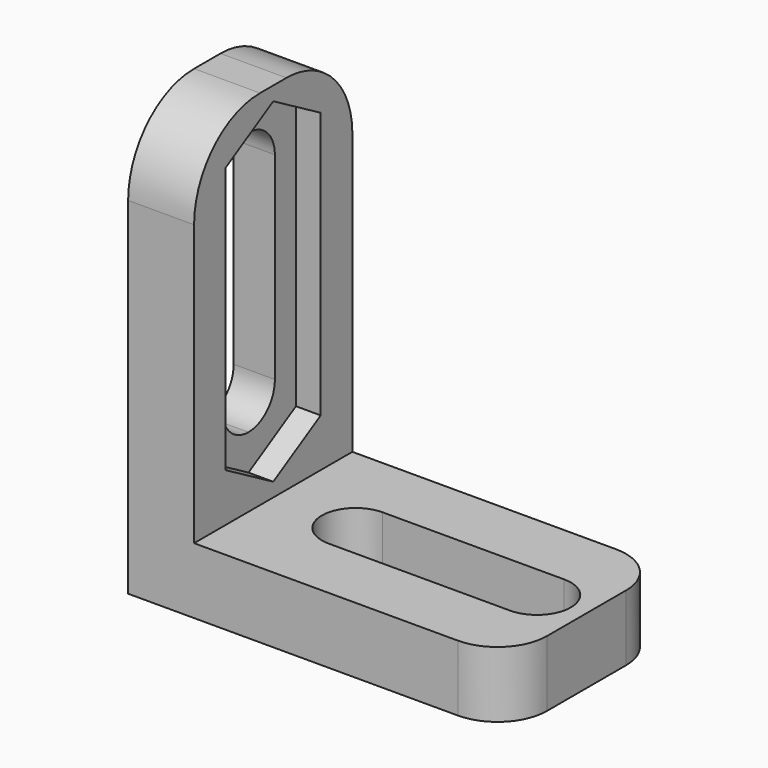
from build123d import *

# Parameters (mm, degrees)
F1_DEPTH = 4
F2_W     = 4
F2_H     = 12
F3_DEPTH = 22
F5_DEPTH = 25
F7_DEPTH = 1.5
F8_R     = 5


# Not quite as in the source:
# - a feature names something its author has since deleted; it is built from what else it names


with BuildPart() as f1:
    # F0 (on Top) → F1 (new body)
    with BuildSketch(Plane.XY):
        with BuildLine():
            ThreePointArc((0, -3), (-0.8786796564, -0.8786796564), (-3, 0))
            Line((-3, 0), (-23, 0))
            Line((-23, 0), (-23, -12))
            Line((-23, -12), (-3, -12))
            ThreePointArc((-3, -12), (-0.8786796564, -11.1213203436), (0, -9))
            Line((0, -9), (0, -3))
        make_face()
        with BuildLine():
            ThreePointArc((-3, -3.95), (-0.95, -6), (-3, -8.05))
            Line((-3, -8.05), (-14, -8.05))
            ThreePointArc((-14, -8.05), (-16.05, -6), (-14, -3.95))
            Line((-14, -3.95), (-3, -3.95))
        make_face(mode=Mode.SUBTRACT)
    extrude(amount=F1_DEPTH)

    # F2 (on face) → F3 (join)
    with BuildSketch(Plane.XY.offset(4)):
        with Locations((-21, -6)):
            Rectangle(F2_W, F2_H)
    extrude(amount=F3_DEPTH)

    # F4 (on face) → F5 (cut)
    with BuildSketch(Plane(origin=(-23, 0, 0), x_dir=(0, -1, 0), z_dir=(-1, 0, 0))):
        with BuildLine():
            Line((4, 21), (4, 9))
            ThreePointArc((4, 9), (4.5857864376, 7.5857864376), (6, 7))
            ThreePointArc((6, 7), (7.4142135624, 7.5857864376), (8, 9))
            Line((8, 9), (8, 21))
            ThreePointArc((8, 21), (7.4142135624, 22.4142135624), (6, 23))
            ThreePointArc((6, 23), (4.5857864376, 22.4142135624), (4, 21))
        make_face()
    extrude(amount=-F5_DEPTH, mode=Mode.SUBTRACT)

    # F6 (on face) → F7 (cut)
    with BuildSketch(Plane.YZ.offset(-19)):
        Polygon((-6, 4.8430780618), (-2.4, 6.9215390309), (-2.4, 23.0784609691), (-6, 25.1569219382), (-9.6, 23.0784609691), (-9.6, 6.9215390309), align=None)
        with BuildLine():
            ThreePointArc((-8, 21), (-6, 23), (-4, 21))
            Line((-4, 21), (-4, 9))
            ThreePointArc((-4, 9), (-6, 7), (-8, 9))
            Line((-8, 9), (-8, 21))
        make_face(mode=Mode.SUBTRACT)
    extrude(amount=-F7_DEPTH, mode=Mode.SUBTRACT)

    # F8
    f8_edges = [f1.edges().sort_by_distance(p)[0] for p in [
        (-21, -12, 26),
        (-21, 0, 26),
    ]]
    fillet(f8_edges, radius=F8_R)


solid = f1.part
